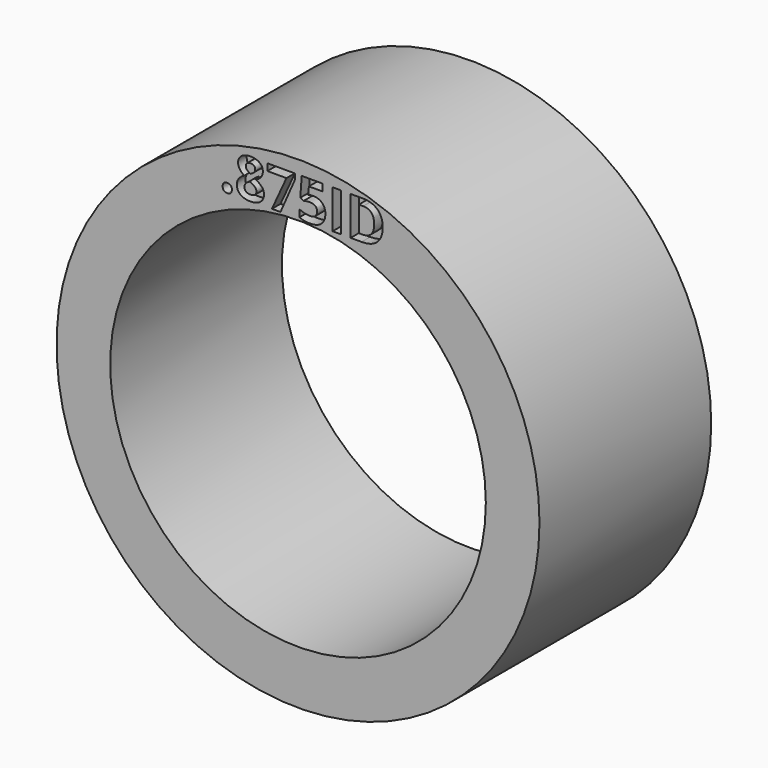
from build123d import *

# Parameters (mm, degrees)
F0_R         = 14.2875
F0_R_2       = 11.1125
F1_DEPTH     = 12.7
F2_TEXT_SIZE = 3.2064804514
F3_DEPTH     = 0.635


# Not quite as in the source:
# - Text() gives the source's letters only with a copy of the font that has no kerning and outlines rounded to 1/6400 em; it was checked with that copy


with BuildPart() as f1:
    # F0 (on Front) → F1 (new body)
    with BuildSketch(Plane.XZ):
        Circle(F0_R)
        Circle(F0_R_2, mode=Mode.SUBTRACT)
    extrude(amount=-F1_DEPTH)

    # F2 (on face) → F3 (cut)
    with BuildSketch(Plane.XZ):
        with Locations((-4.6432157652, 11.2032992765)):
            Text('.875ID', F2_TEXT_SIZE, font='Open Sans', font_style=FontStyle.BOLD, text_align=(TextAlign.LEFT, TextAlign.BOTTOM))
    extrude(amount=-F3_DEPTH, mode=Mode.SUBTRACT)


solid = f1.part
